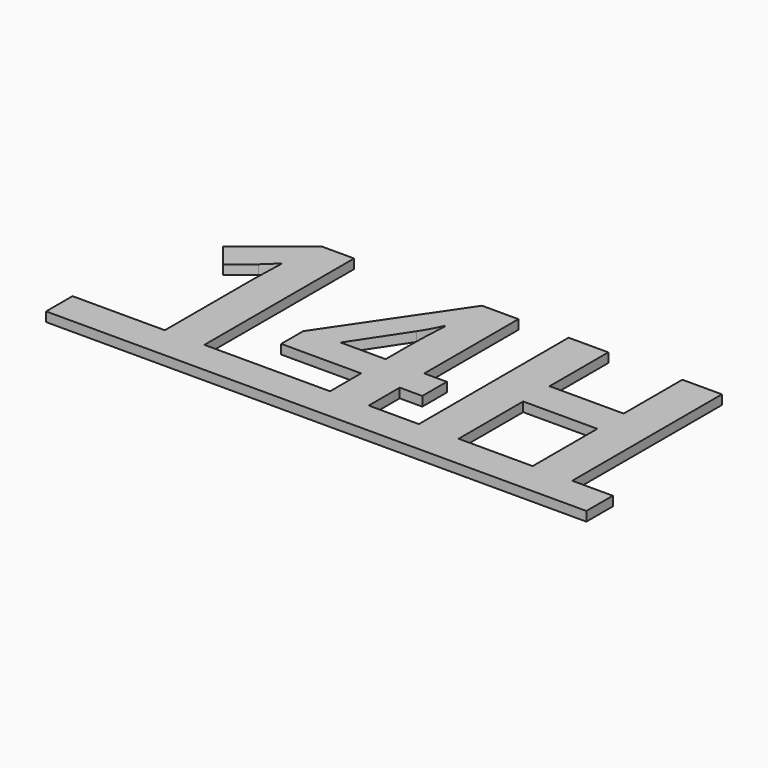
from build123d import *

# Parameters (mm, degrees)
F0_TEXT_SIZE = 1411.1111111111
F1_DEPTH     = 50.8


# Not quite as in the source:
# - a feature names something its author has since deleted; it is built from what else it names
# - Text() gives the source's letters only with a copy of the font that has no kerning and outlines rounded to 1/6400 em; it was checked with that copy


with BuildPart() as f1:
    # F0 (on Top) → F1 (new body)
    with BuildSketch(Plane.XY):
        Polygon((-281.1885137558, 0), (-281.1885137558, -177.8), (2627.464264022, -177.8), (2627.464264022, 0), (2408.9625279109, 0), (2195.9729445775, 0), (1797.1135695775, 0), (1583.4625279109, 0), (1313.3670417998, 0), (1105.2281529109, 0), (428.776764022, 0), (215.7871806886, 0), align=None)
        with Locations((-154.1885137558, 0)):
            Text('14H', F0_TEXT_SIZE, font='Open Sans', font_style=FontStyle.BOLD, text_align=(TextAlign.LEFT, TextAlign.BOTTOM))
    extrude(amount=F1_DEPTH)


solid = f1.part
